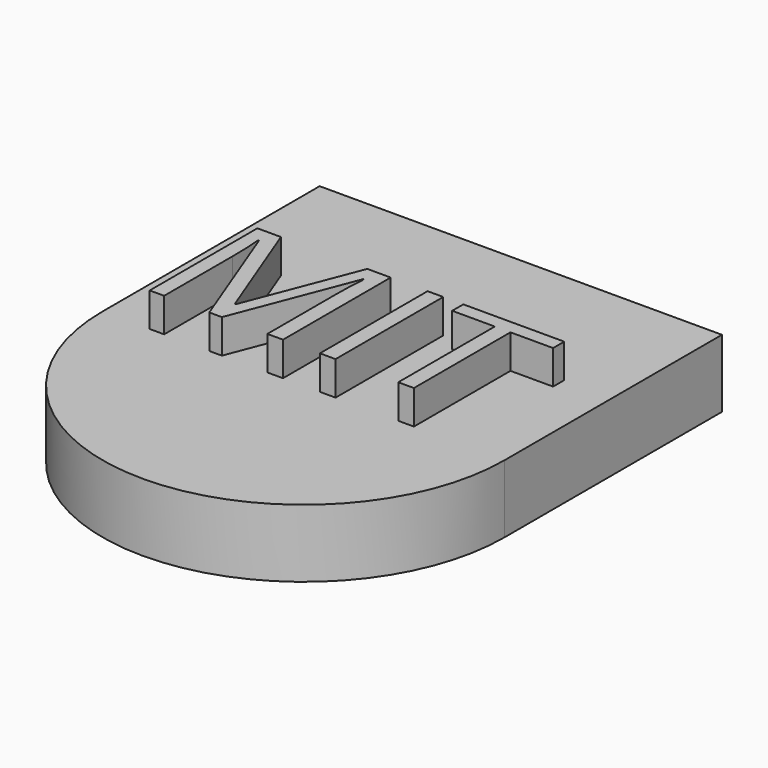
from build123d import *

# Parameters (mm, degrees)
F1_DEPTH     = 25.4
F2_TEXT_SIZE = 70.5555555556
F3_DEPTH     = 12.7


# Not quite as in the source:
# - Text() gives the source's letters only with a copy of the font that has no kerning and outlines rounded to 1/6400 em; it was checked with that copy


with BuildPart() as f1:
    # F0 (on Top) → F1 (new body)
    with BuildSketch(Plane.XY):
        with BuildLine():
            Line((-75.2676250473, 101.6), (-75.2676250473, 0))
            ThreePointArc((-75.2676250473, 0), (0, -75.2676250473), (75.2676250473, 0))
            Line((75.2676250473, 0), (75.2676250473, 101.6))
            Line((75.2676250473, 101.6), (-75.2676250473, 101.6))
        make_face()
    extrude(amount=F1_DEPTH)

    # F2 (on face) → F3 (join)
    with BuildSketch(Plane.XY.offset(25.4)):
        with Locations((-64.5035548417, 0)):
            Text('MIT', F2_TEXT_SIZE, font='Open Sans', text_align=(TextAlign.LEFT, TextAlign.BOTTOM))
    extrude(amount=F3_DEPTH)


solid = f1.part
